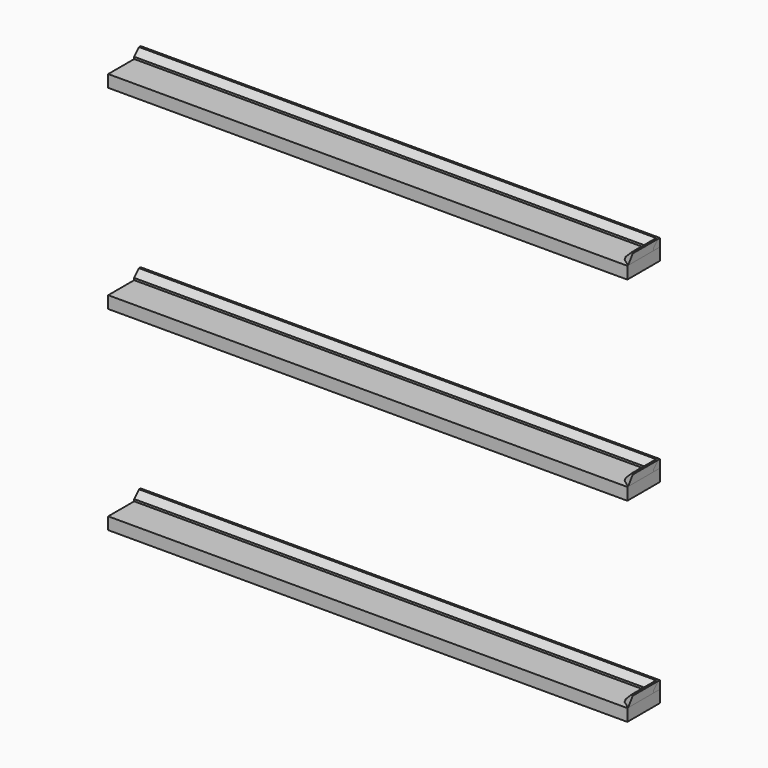
from build123d import *

# Parameters (mm, degrees)
F2_W          = 812.8
F2_H          = 19.05
F3_DEPTH      = 63.5
F5_DEPTH      = 63.5
F6_T1_DEPTH   = 78.7911320759
F6_2_T1_DEPTH = 78.7911320759
F6_3_T1_DEPTH = 78.7911320759
F8_DEPTH      = 25.4
F8_DEPTH_BACK = 762
F10_DEPTH     = 812.8


# Not quite as in the source:
# - a fillet or chamfer that OpenCascade refuses, or shapes differently, is made with other operations: its cross-section is extruded or revolved along the edge and cut away or added


with BuildPart() as f3:
    # F2 (on face) → F3 (new body)
    with BuildSketch(Plane.XZ.offset(-76.2)):
        with Locations((16.8031001225, 1362.075)):
            Rectangle(F2_W, F2_H)
    extrude(amount=F3_DEPTH)


with BuildPart() as f3b:
    # F2 (on face) → F3, piece 2 (new body)
    with BuildSketch(Plane.XZ.offset(-76.2)):
        with Locations((16.8031001225, 1057.275)):
            Rectangle(F2_W, F2_H)
    extrude(amount=F3_DEPTH)


with BuildPart() as f3c:
    # F2 (on face) → F3, piece 3 (new body)
    with BuildSketch(Plane.XZ.offset(-76.2)):
        with Locations((16.8031001225, 752.475)):
            Rectangle(F2_W, F2_H)
    extrude(amount=F3_DEPTH)


with BuildPart() as f5:
    # F4 (on face) → F5 (new body)
    with BuildSketch(Plane.XZ.offset(-76.2)):
        Polygon((410.5031001225, 1371.6), (423.2031001225, 1371.6), (423.2031001225, 1384.3), (420.0281001225, 1384.3), (410.5031001225, 1374.775), align=None)
    extrude(amount=F5_DEPTH)

    # F6: chamfer of 12.7 on 1 edges, made by hand

    # F6_s2 → F6_t1 (cut)
    with BuildSketch(Plane(origin=(925.2584219554, 0, 925.2584219554), x_dir=(0, 1, 0), z_dir=(-0.7071067812, 0, -0.7071067812))):
        Polygon((25.4, -681.843199311), (12.7, -669.143199311), (12.7, -681.843199311), align=None)
    extrude(amount=F6_T1_DEPTH, mode=Mode.SUBTRACT)


with BuildPart() as f5b:
    # F4 (on face) → F5, piece 2 (new body)
    with BuildSketch(Plane.XZ.offset(-76.2)):
        Polygon((410.5031001225, 1066.8), (423.2031001225, 1066.8), (423.2031001225, 1079.5), (420.0281001225, 1079.5), (410.5031001225, 1069.975), align=None)
    extrude(amount=F5_DEPTH)

    # F6#2: chamfer of 12.7 on 1 edges, made by hand

    # F6_2_s2 → F6_2_t1 (cut)
    with BuildSketch(Plane(origin=(772.8584219554, 0, 772.8584219554), x_dir=(0, 1, 0), z_dir=(-0.7071067812, 0, -0.7071067812))):
        Polygon((25.4, -466.3170524054), (12.7, -453.6170524054), (12.7, -466.3170524054), align=None)
    extrude(amount=F6_2_T1_DEPTH, mode=Mode.SUBTRACT)


with BuildPart() as f5c:
    # F4 (on face) → F5, piece 3 (new body)
    with BuildSketch(Plane.XZ.offset(-76.2)):
        Polygon((410.5031001225, 762), (423.2031001225, 762), (423.2031001225, 774.7), (420.0281001225, 774.7), (410.5031001225, 765.175), align=None)
    extrude(amount=F5_DEPTH)

    # F6#3: chamfer of 12.7 on 1 edges, made by hand

    # F6_3_s2 → F6_3_t1 (cut)
    with BuildSketch(Plane(origin=(620.4584219554, 0, 620.4584219554), x_dir=(0, 1, 0), z_dir=(-0.7071067812, 0, -0.7071067812))):
        Polygon((25.4, -250.7909054997), (12.7, -238.0909054997), (12.7, -250.7909054997), align=None)
    extrude(amount=F6_3_T1_DEPTH, mode=Mode.SUBTRACT)


with BuildPart() as f8_tool:
    # F7 (on face) → F8 (new body, two sides)
    with BuildSketch(Plane.XY.offset(1371.6)) as f8_sk:
        Polygon((405.7026830367, 58.6995829142), (423.2031001225, 76.2), (423.2031001225, 80.5244233704), (405.7026830367, 80.5244233704), align=None)
    extrude(amount=F8_DEPTH)
    extrude(f8_sk.sketch, amount=-F8_DEPTH_BACK)


with BuildPart() as f5_1:
    add(f5.part)

    # F8: cut by f8_tool
    add(f8_tool.part, mode=Mode.SUBTRACT)


with BuildPart() as f5b_1:
    add(f5b.part)

    # F8: cut by f8_tool
    add(f8_tool.part, mode=Mode.SUBTRACT)


with BuildPart() as f5c_1:
    add(f5c.part)

    # F8: cut by f8_tool
    add(f8_tool.part, mode=Mode.SUBTRACT)


with BuildPart() as f10:
    # F9 (on face) → F10 (new body)
    with BuildSketch(Plane(origin=(423.2031001225, 0, 0), x_dir=(0, -1, 0), z_dir=(-1, 0, 0))):
        Polygon((-76.2, 1384.3), (-76.2, 1371.6), (-63.5, 1371.6), (-63.5, 1374.775), (-73.025, 1384.3), align=None)
    extrude(amount=F10_DEPTH)


with BuildPart() as f10b:
    # F9 (on face) → F10, piece 2 (new body)
    with BuildSketch(Plane(origin=(423.2031001225, 0, 0), x_dir=(0, -1, 0), z_dir=(-1, 0, 0))):
        Polygon((-76.2, 1079.5), (-76.2, 1066.8), (-63.5, 1066.8), (-63.5, 1069.975), (-73.025, 1079.5), align=None)
    extrude(amount=F10_DEPTH)


with BuildPart() as f10c:
    # F9 (on face) → F10, piece 3 (new body)
    with BuildSketch(Plane(origin=(423.2031001225, 0, 0), x_dir=(0, -1, 0), z_dir=(-1, 0, 0))):
        Polygon((-76.2, 774.7), (-76.2, 762), (-63.5, 762), (-63.5, 765.175), (-73.025, 774.7), align=None)
    extrude(amount=F10_DEPTH)


solid = Compound([f3.part, f3b.part, f3c.part, f5_1.part, f5b_1.part, f5c_1.part, f10.part, f10b.part, f10c.part])
